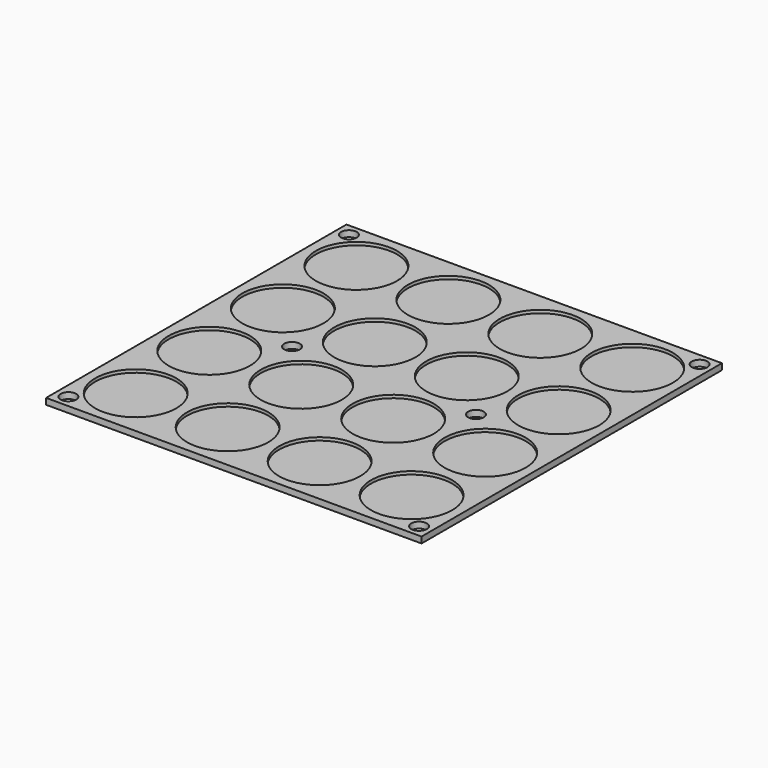
from build123d import *

# Parameters (mm, degrees)
F0_W     = 122.5
F0_H     = 122.5
F0_R     = 13.25
F1_DEPTH = 1
F2_DEPTH = 2
F3_R     = 2.55
F4_DEPTH = 2.001


# Not quite as in the source:
# - a feature names something its author has since deleted; it is built from what else it names


with BuildPart() as f1:
    # F0 (on Top) → F1 (new body)
    with BuildSketch(Plane.XY):
        Rectangle(F0_W, F0_H)
        with Locations((-45, -45)):
            Circle(F0_R, mode=Mode.SUBTRACT)
        with Locations((-15, -45)):
            Circle(F0_R, mode=Mode.SUBTRACT)
        with Locations((-45, -15)):
            Circle(F0_R, mode=Mode.SUBTRACT)
        with Locations((-15, -15)):
            Circle(F0_R, mode=Mode.SUBTRACT)
        with Locations((15, -45)):
            Circle(F0_R, mode=Mode.SUBTRACT)
        with Locations((45, -45)):
            Circle(F0_R, mode=Mode.SUBTRACT)
        with Locations((15, -15)):
            Circle(F0_R, mode=Mode.SUBTRACT)
        with Locations((45, -15)):
            Circle(F0_R, mode=Mode.SUBTRACT)
        with Locations((-45, 15)):
            Circle(F0_R, mode=Mode.SUBTRACT)
        with Locations((-15, 15)):
            Circle(F0_R, mode=Mode.SUBTRACT)
        with Locations((-45, 45)):
            Circle(F0_R, mode=Mode.SUBTRACT)
        with Locations((-15, 45)):
            Circle(F0_R, mode=Mode.SUBTRACT)
        with Locations((15, 15)):
            Circle(F0_R, mode=Mode.SUBTRACT)
        with Locations((45, 15)):
            Circle(F0_R, mode=Mode.SUBTRACT)
        with Locations((15, 45)):
            Circle(F0_R, mode=Mode.SUBTRACT)
        with Locations((45, 45)):
            Circle(F0_R, mode=Mode.SUBTRACT)
        with Locations((-45, 45)):
            Circle(F0_R)
        with Locations((-15, 45)):
            Circle(F0_R)
        with Locations((15, 45)):
            Circle(F0_R)
        with Locations((45, 45)):
            Circle(F0_R)
        with Locations((45, 15)):
            Circle(F0_R)
        with Locations((-15, 15)):
            Circle(F0_R)
        with Locations((-45, 15)):
            Circle(F0_R)
        with Locations((15, 15)):
            Circle(F0_R)
        with Locations((15, -15)):
            Circle(F0_R)
        with Locations((-15, -15)):
            Circle(F0_R)
        with Locations((-45, -15)):
            Circle(F0_R)
        with Locations((45, -15)):
            Circle(F0_R)
        with Locations((45, -45)):
            Circle(F0_R)
        with Locations((15, -45)):
            Circle(F0_R)
        with Locations((-15, -45)):
            Circle(F0_R)
        with Locations((-45, -45)):
            Circle(F0_R)
    extrude(amount=F1_DEPTH)

    # F0 (on Top) → F2 (join)
    with BuildSketch(Plane.XY):
        Rectangle(F0_W, F0_H)
        with Locations((-45, -45)):
            Circle(F0_R, mode=Mode.SUBTRACT)
        with Locations((-15, -45)):
            Circle(F0_R, mode=Mode.SUBTRACT)
        with Locations((-45, -15)):
            Circle(F0_R, mode=Mode.SUBTRACT)
        with Locations((-15, -15)):
            Circle(F0_R, mode=Mode.SUBTRACT)
        with Locations((15, -45)):
            Circle(F0_R, mode=Mode.SUBTRACT)
        with Locations((45, -45)):
            Circle(F0_R, mode=Mode.SUBTRACT)
        with Locations((15, -15)):
            Circle(F0_R, mode=Mode.SUBTRACT)
        with Locations((45, -15)):
            Circle(F0_R, mode=Mode.SUBTRACT)
        with Locations((-45, 15)):
            Circle(F0_R, mode=Mode.SUBTRACT)
        with Locations((-15, 15)):
            Circle(F0_R, mode=Mode.SUBTRACT)
        with Locations((-45, 45)):
            Circle(F0_R, mode=Mode.SUBTRACT)
        with Locations((-15, 45)):
            Circle(F0_R, mode=Mode.SUBTRACT)
        with Locations((15, 15)):
            Circle(F0_R, mode=Mode.SUBTRACT)
        with Locations((45, 15)):
            Circle(F0_R, mode=Mode.SUBTRACT)
        with Locations((15, 45)):
            Circle(F0_R, mode=Mode.SUBTRACT)
        with Locations((45, 45)):
            Circle(F0_R, mode=Mode.SUBTRACT)
    extrude(amount=F2_DEPTH)

    # F3 (on face) → F4 (cut, through all)
    with BuildSketch(Plane.XY.offset(2)):
        with Locations((-57.2, 57.2)):
            Circle(F3_R)
        with Locations((-30, 0)):
            Circle(F3_R)
        with Locations((57.2, 57.2)):
            Circle(F3_R)
        with Locations((30, 0)):
            Circle(F3_R)
        with Locations((57.2, -57.2)):
            Circle(F3_R)
        with Locations((-57.2, -57.2)):
            Circle(F3_R)
    extrude(amount=-F4_DEPTH, mode=Mode.SUBTRACT)


solid = f1.part
